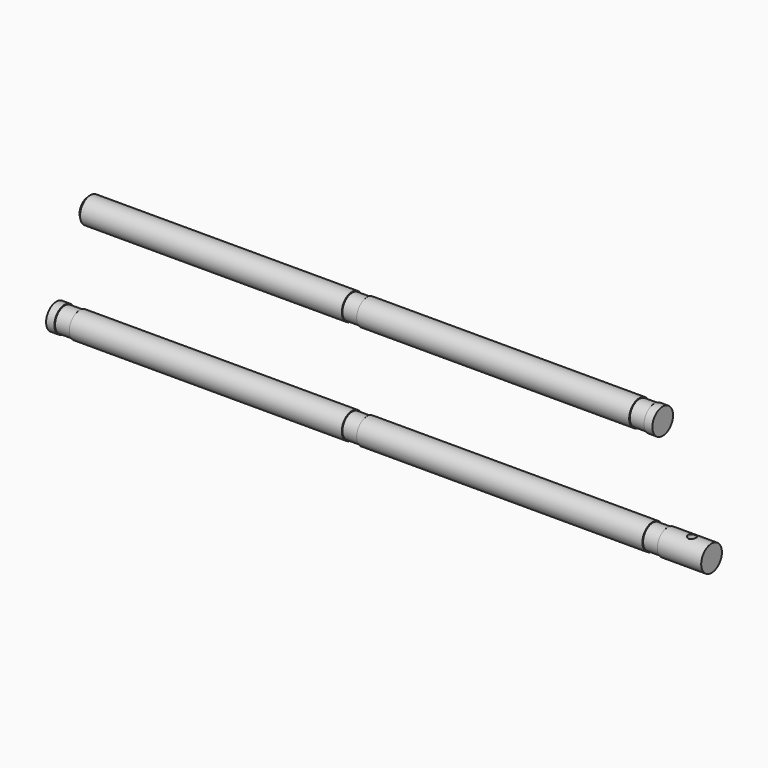
from build123d import *

# Parameters (mm, degrees)
F0_R           = 3.7211
F1_DEPTH       = 2.286
F1_DEPTH_BACK  = 2.286
F2_R           = 3.96875
F2_R_2         = 3.7211
F3_DEPTH       = 87.63
F4_R           = 3.7211
F5_DEPTH       = 4.572
F6_R           = 3.96875
F6_R_2         = 3.7211
F7_DEPTH       = 13.462
F8_R           = 3.96875
F8_R_2         = 3.7211
F9_DEPTH       = 83.566
F10_R          = 3.7211
F11_DEPTH      = 4.572
F12_R          = 3.96875
F12_R_2        = 3.7211
F13_DEPTH      = 2.54
F16_R          = 1.2192
F17_DEPTH      = 25.4
F18_R          = 3.7211
F19_DEPTH      = 2.286
F19_DEPTH_BACK = 2.286
F20_R          = 3.96875
F20_R_2        = 3.7211
F21_DEPTH      = 83.566
F22_R          = 3.7211
F23_DEPTH      = 4.572
F24_R          = 3.96875
F24_R_2        = 3.7211
F25_DEPTH      = 2.54
F26_R          = 3.96875
F26_R_2        = 3.7211
F27_DEPTH      = 81.026
F28_SIZE       = 0.762


with BuildPart() as f1:
    # F0 (on Right) → F1 (new body, two sides)
    with BuildSketch(Plane.YZ) as f1_sk:
        Circle(F0_R)
    extrude(amount=F1_DEPTH)
    extrude(f1_sk.sketch, amount=-F1_DEPTH_BACK)

    # F2 (on face) → F3 (join)
    with BuildSketch(Plane.YZ.offset(2.286)):
        Circle(F2_R)
        Circle(F2_R_2, mode=Mode.SUBTRACT)
        Circle(F2_R_2)
    extrude(amount=F3_DEPTH)

    # F4 (on face) → F5 (join)
    with BuildSketch(Plane.YZ.offset(89.916)):
        Circle(F4_R)
    extrude(amount=F5_DEPTH)

    # F6 (on face) → F7 (join)
    with BuildSketch(Plane.YZ.offset(94.488)):
        Circle(F6_R)
        Circle(F6_R_2, mode=Mode.SUBTRACT)
        Circle(F6_R_2)
    extrude(amount=F7_DEPTH)

    # F8 (on face) → F9 (join)
    with BuildSketch(Plane(origin=(-2.286, 0, 0), x_dir=(0, -1, 0), z_dir=(-1, 0, 0))):
        Circle(F8_R)
        Circle(F8_R_2, mode=Mode.SUBTRACT)
        Circle(F8_R_2)
    extrude(amount=F9_DEPTH)

    # F10 (on face) → F11 (join)
    with BuildSketch(Plane(origin=(-85.852, 0, 0), x_dir=(0, -1, 0), z_dir=(-1, 0, 0))):
        Circle(F10_R)
    extrude(amount=F11_DEPTH)

    # F12 (on face) → F13 (join)
    with BuildSketch(Plane(origin=(-90.424, 0, 0), x_dir=(0, -1, 0), z_dir=(-1, 0, 0))):
        Circle(F12_R)
        Circle(F12_R_2, mode=Mode.SUBTRACT)
        Circle(F12_R_2)
    extrude(amount=F13_DEPTH)

    # F16 (on plane+point) → F17 (cut)
    with BuildSketch(Plane.XY.offset(3.96875)):
        with Locations((101.9604578614, 0)):
            Circle(F16_R)
    extrude(amount=-F17_DEPTH, mode=Mode.SUBTRACT)


with BuildPart() as f19:
    # F18 (on Right) → F19 (new body, two sides)
    with BuildSketch(Plane.YZ) as f19_sk:
        with Locations((0, 32.1224965155)):
            Circle(F18_R)
    extrude(amount=F19_DEPTH)
    extrude(f19_sk.sketch, amount=-F19_DEPTH_BACK)

    # F20 (on face) → F21 (join)
    with BuildSketch(Plane.YZ.offset(2.286)):
        with Locations((0, 32.1224965155)):
            Circle(F20_R)
        with Locations((0, 32.1224965155)):
            Circle(F20_R_2, mode=Mode.SUBTRACT)
        with Locations((0, 32.1224965155)):
            Circle(F20_R_2)
    extrude(amount=F21_DEPTH)

    # F22 (on face) → F23 (join)
    with BuildSketch(Plane.YZ.offset(85.852)):
        with Locations((0, 32.1224965155)):
            Circle(F22_R)
    extrude(amount=F23_DEPTH)

    # F24 (on face) → F25 (join)
    with BuildSketch(Plane.YZ.offset(90.424)):
        with Locations((0, 32.1224965155)):
            Circle(F24_R)
        with Locations((0, 32.1224965155)):
            Circle(F24_R_2, mode=Mode.SUBTRACT)
        with Locations((0, 32.1224965155)):
            Circle(F24_R_2)
    extrude(amount=F25_DEPTH)

    # F26 (on face) → F27 (join)
    with BuildSketch(Plane(origin=(-2.286, 0, 0), x_dir=(0, -1, 0), z_dir=(-1, 0, 0))):
        with Locations((0, 32.1224965155)):
            Circle(F26_R)
        with Locations((0, 32.1224965155)):
            Circle(F26_R_2, mode=Mode.SUBTRACT)
        with Locations((0, 32.1224965155)):
            Circle(F26_R_2)
    extrude(amount=F27_DEPTH)

    # F28
    f28_edges = [f19.edges().sort_by_distance(p)[0] for p in [
        (-83.312, 3.96875, 32.122497),
    ]]
    chamfer(f28_edges, length=F28_SIZE)


solid = Compound([f1.part, f19.part])
